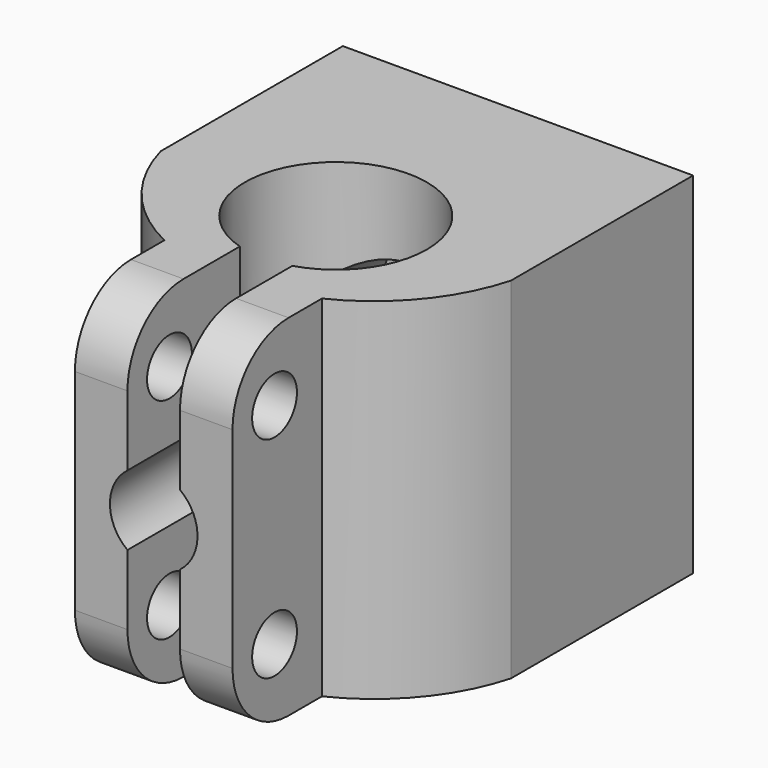
from build123d import *

# Parameters (mm, degrees)
F1_DEPTH = 10
F3_D     = 5
F4_R     = 1.6
F5_DEPTH = 14.501
F7_R     = 5.5
F8_DEPTH = 10
F9_R     = 4


# Not quite as in the source:
# - an extrude ends at something that could not be found from the text; its depth is read off the source's solid


with BuildPart() as f1:
    # F0 (on Top) → F1 (new body, symmetric)
    with BuildSketch(Plane.XY):
        with BuildLine():
            Line((10, 13), (-10, 13))
            Line((-10, 13), (-10, 0))
            ThreePointArc((-10, 0), (-7.9686887253, -3.9047945105), (-4.5, -6.6143782777))
            Line((-4.5, -6.6143782777), (-4.5, -13))
            Line((-4.5, -13), (-1.5, -13))
            Line((-1.5, -13), (-1.5, -4.9789557138))
            ThreePointArc((-1.5, -4.9789557138), (-3.1016124839, 4.1737273509), (5.2, 0))
            ThreePointArc((5.2, 0), (4.1737273509, -3.1016124839), (1.5, -4.9789557138))
            Line((1.5, -4.9789557138), (1.5, -13))
            Line((1.5, -13), (4.5, -13))
            Line((4.5, -13), (4.5, -6.6143782777))
            ThreePointArc((4.5, -6.6143782777), (7.9686887253, -3.9047945105), (10, 0))
            Line((10, 0), (10, 13))
        make_face()
    extrude(amount=F1_DEPTH, both=True)

    # F3 (through all)
    with Locations(Plane(origin=(0, 13, 0), x_dir=(-1, 0, 0), z_dir=(0, 1, 0))):
        with Locations((0, 0)):
            Hole(F3_D / 2)

    # F4 (on face) → F5 (cut, through all)
    with BuildSketch(Plane(origin=(-4.5, 0, 0), x_dir=(0, -1, 0), z_dir=(-1, 0, 0))):
        with Locations((10, 6)):
            Circle(F4_R)
        with Locations((10, -6)):
            Circle(F4_R)
    extrude(amount=-F5_DEPTH, mode=Mode.SUBTRACT)

    # F7 (on offset) → F8 (cut, through all)
    with BuildSketch(Plane.XZ.offset(-10)):
        Circle(F7_R)
    extrude(amount=F8_DEPTH, mode=Mode.SUBTRACT)

    # F9
    f9_edges = [f1.edges().sort_by_distance(p)[0] for p in [
        (3, -13, 10),
        (-3, -13, 10),
        (-3, -13, -10),
        (3, -13, -10),
    ]]
    fillet(f9_edges, radius=F9_R)


solid = f1.part
